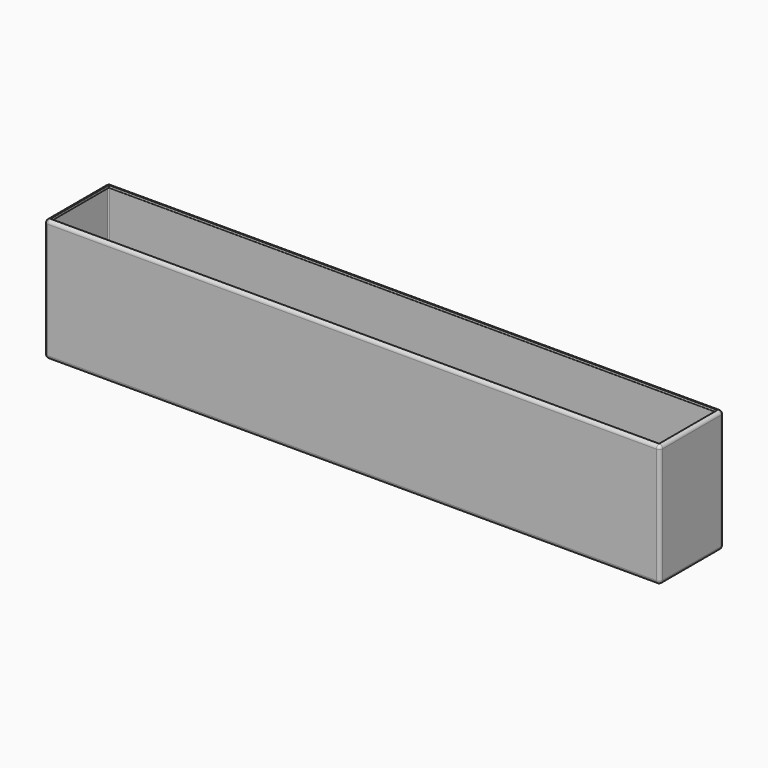
from build123d import *

# Parameters (mm, degrees)
F0_W     = 685.8
F0_H     = 136.525
F1_DEPTH = 88.9
F2_R     = 3.81
F3_T     = -2.54


# Not quite as in the source:
# - a shell that OpenCascade refuses in one call is made with other operations: the cavity is built on its own and cut out


with BuildPart() as f1:
    # F0 (on Front) → F1 (new body)
    with BuildSketch(Plane.XZ):
        Rectangle(F0_W, F0_H)
    extrude(amount=F1_DEPTH)

    # F2
    f2_edges = [f1.edges().sort_by_distance(p)[0] for p in [
        (-342.9, -44.45, 68.2625),
        (342.9, -44.45, 68.2625),
        (0, 0, 68.2625),
        (0, -88.9, 68.2625),
        (-342.9, 0, 0),
        (0, 0, -68.2625),
        (342.9, 0, 0),
        (-342.9, -44.45, -68.2625),
        (-342.9, -88.9, 0),
        (0, -88.9, -68.2625),
        (342.9, -88.9, 0),
        (342.9, -44.45, -68.2625),
    ]]
    fillet(f2_edges, radius=F2_R)

    # F3: a shell. OpenCascade refuses it in one call, so the cavity is built on its own and cut out:
    # the body offset inwards by the wall thickness, plus a prism from it out through each open face.
    f3_core = offset(f1.part, amount=F3_T, mode=Mode.PRIVATE)
    f3_exits = [f3_core.faces().sort_by_distance(p)[0] for p in [
        (0, -44.45, 65.7225),
    ]]
    add(f3_core, mode=Mode.SUBTRACT)
    extrude(f3_exits, amount=-F3_T, mode=Mode.SUBTRACT)


solid = f1.part
